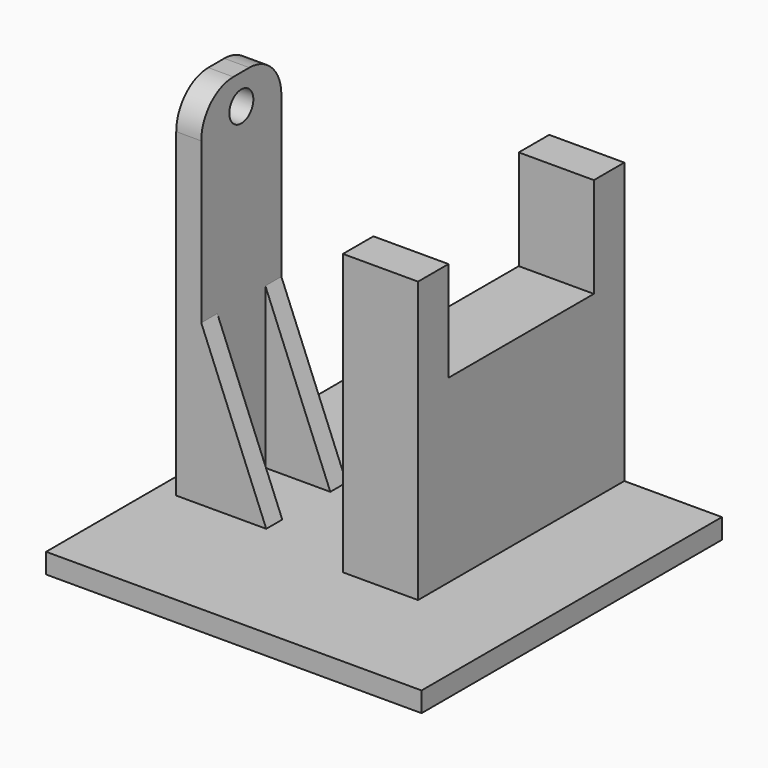
from build123d import *

# Parameters (mm, degrees)
F0_W      = 47.625
F0_H      = 47.625
F1_DEPTH  = 2.54
F3_W      = 9.525
F3_H      = 32.7025
F4_DEPTH  = 22.86
F5_W      = 9.525
F5_H      = 4.826
F6_DEPTH  = 12.7
F7_W      = 3.175
F7_H      = 12.7
F8_DEPTH  = 45.72
F9_R      = 1.905
F10_DEPTH = 25.4
F11_R     = 5.08
F13_DEPTH = 2.54


# Not quite as in the source:
# - a pattern or mirror of a feature is missing from the dataset's text; its kind, count and spacing are read off the source's solid


with BuildPart() as f1:
    # F0 (on Top) → F1 (new body)
    with BuildSketch(Plane.XY):
        Rectangle(F0_W, F0_H)
    extrude(amount=F1_DEPTH)

    # F3 (on face) → F4 (join)
    with BuildSketch(Plane.XY.offset(2.54)):
        with Locations((6.6675, 7.46125)):
            Rectangle(F3_W, F3_H)
    extrude(amount=F4_DEPTH)

    # F5 (on face) → F6 (join)
    with BuildSketch(Plane.XY.offset(25.4)):
        with Locations((6.6675, -6.477)):
            Rectangle(F5_W, F5_H)
        with Locations((6.6675, 21.3995)):
            Rectangle(F5_W, F5_H)
    extrude(amount=F6_DEPTH)

    # F7 (on face) → F8 (join)
    with BuildSketch(Plane.XY.offset(2.54)):
        with Locations((-19.685, 0)):
            Rectangle(F7_W, F7_H)
    extrude(amount=F8_DEPTH)

    # F9 (on face) → F10 (cut)
    with BuildSketch(Plane.YZ.offset(-18.0975)):
        with Locations((0, 44.45)):
            Circle(F9_R)
    extrude(amount=-F10_DEPTH, mode=Mode.SUBTRACT)

    # F11
    f11_edges = [f1.edges().sort_by_distance(p)[0] for p in [
        (-19.685, 6.35, 48.26),
        (-19.685, -6.35, 48.26),
    ]]
    fillet(f11_edges, radius=F11_R)

    # F12 (on face) → F13 (join)
    with BuildSketch(Plane(origin=(0, 6.35, 0), x_dir=(-1, 0, 0), z_dir=(0, 1, 0))):
        Polygon((18.0975, 2.54), (18.0975, 22.86), (9.8562051214, 2.54), align=None)
    f13 = extrude(amount=-F13_DEPTH)

    # F13_copies: F13 across plane
    add(f13.mirror(Plane(origin=(0, 0, 0), x_dir=(0, 0, -1), z_dir=(0, -1, 0))))


solid = f1.part
